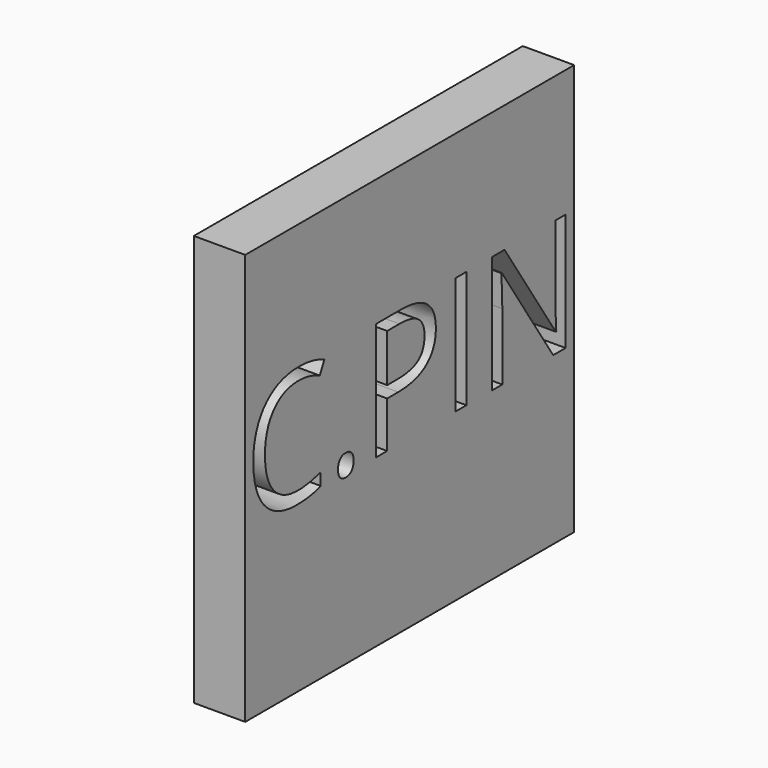
from build123d import *

# Parameters (mm, degrees)
F0_W         = 101.6
F0_H         = 101.6
F1_DEPTH     = 12.7
F2_TEXT_SIZE = 40.6654158849
F3_DEPTH     = 25


# Not quite as in the source:
# - Text() gives the source's letters only with a copy of the font that has no kerning and outlines rounded to 1/6400 em; it was checked with that copy


with BuildPart() as f1:
    # F0 (on Right) → F1 (new body)
    with BuildSketch(Plane.YZ):
        with Locations((-3.2078959048, 9.2667647884)):
            Rectangle(F0_W, F0_H)
    extrude(amount=F1_DEPTH)

    # F2 (on face) → F3 (cut)
    with BuildSketch(Plane.YZ.offset(12.7)):
        with Locations((-54.0078959048, -0.4089417665)):
            Text('C.PIN', F2_TEXT_SIZE, font='Open Sans', text_align=(TextAlign.LEFT, TextAlign.BOTTOM))
    extrude(amount=-F3_DEPTH, mode=Mode.SUBTRACT)


solid = f1.part
